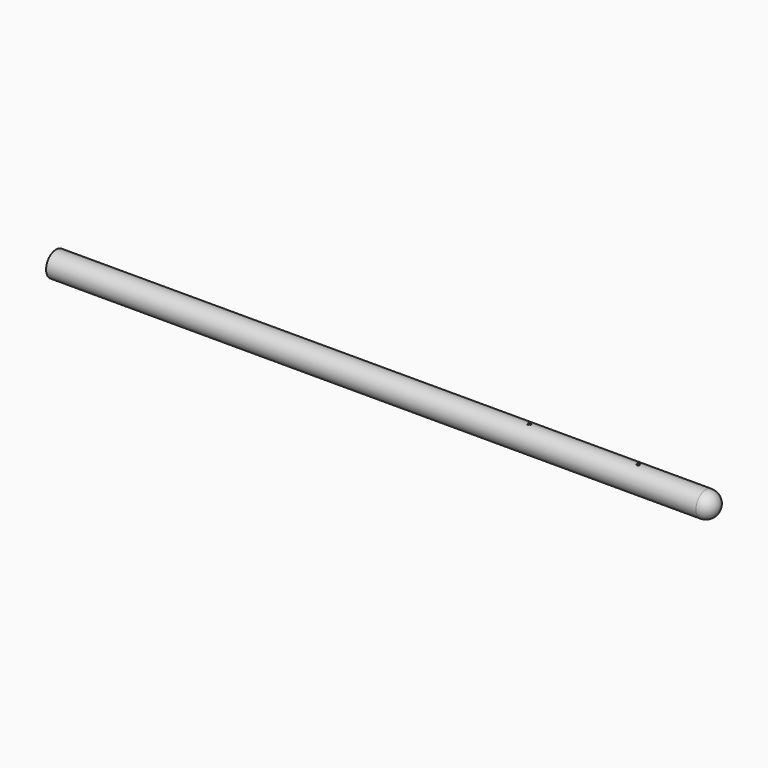
from build123d import *

# Parameters (mm, degrees)
F2_T      = -12.7
F3_R      = 50.8
F4_DEPTH  = 254
F5_DEPTH  = 25.4
F6_R      = 12.7
F7_DEPTH  = 304.8
F9_R      = 15.0991229188
F9_R_2    = 6.35
F9_R_3    = 14.3550520621
F10_DEPTH = 12.7
F11_R     = 5.08
F12_SIZE  = 1.27
F13_R     = 5.08


with BuildPart() as f1:
    # F0 (on Front) → F1 (revolve)
    with BuildSketch(Plane.XZ):
        with BuildLine():
            Line((0, 152.4), (0, 0))
            Line((0, 0), (7924.8, 0))
            Line((7924.8, 0), (8077.2, 0))
            ThreePointArc((8077.2, 0), (8032.5630734528, 107.7630734528), (7924.8, 152.4))
            Line((7924.8, 152.4), (0, 152.4))
        make_face()
    revolve(axis=Axis((4038.6, 0, 0), (1, 0, 0)))

    # F2
    f2_openings = [f1.faces().sort_by_distance(p)[0] for p in [
        (0, 0, 0),
    ]]
    offset(amount=F2_T, openings=f2_openings)

    # F3 (on Top) → F4 (cut)
    with BuildSketch(Plane.XY):
        with Locations((7620, 0)):
            Circle(F3_R)
        with Locations((6096, 0)):
            Circle(F3_R)
        with Locations((4572, 0)):
            Circle(F3_R)
        with Locations((3048, 0)):
            Circle(F3_R)
        with Locations((1524, 0)):
            Circle(F3_R)
    extrude(amount=-F4_DEPTH, mode=Mode.SUBTRACT)

    # F6 (on Top) → F7 (cut)
    with BuildSketch(Plane.XY):
        with Locations((7100.4438400269, 0)):
            Circle(F6_R)
        with Locations((5773.1170654297, 0)):
            Circle(F6_R)
    extrude(amount=F7_DEPTH, mode=Mode.SUBTRACT)

    # F9 (on offset) → F10 (join, symmetric)
    with BuildSketch(Plane.XY.offset(152.4)):
        with Locations((5772.6697921753, 0)):
            Circle(F9_R)
        with Locations((5772.6697921753, 0)):
            Circle(F9_R_2, mode=Mode.SUBTRACT)
        with Locations((7100.5816459656, 0)):
            Circle(F9_R_3)
        with Locations((7100.5816459656, 0)):
            Circle(F9_R_2, mode=Mode.SUBTRACT)
    extrude(amount=F10_DEPTH, both=True)

    # F11
    f11_edges = [f1.edges().sort_by_distance(p)[0] for p in [
        (7100.581646, -14.355052, 151.722419),
        (7100.581646, 14.355052, 151.722419),
    ]]
    fillet(f11_edges, radius=F11_R)

    # F12
    f12_edges = [f1.edges().sort_by_distance(p)[0] for p in [
        (7086.226594, 0, 165.1),
        (5757.570669, 0, 165.1),
    ]]
    chamfer(f12_edges, length=F12_SIZE)

    # F13
    f13_edges = [f1.edges().sort_by_distance(p)[0] for p in [
        (5772.669792, -15.099123, 151.650178),
        (5772.669792, 15.099123, 151.650178),
    ]]
    fillet(f13_edges, radius=F13_R)


with BuildPart() as f5:
    # F3 (on Top) → F5 (new body)
    with BuildSketch(Plane.XY):
        with Locations((7620, 0)):
            Circle(F3_R)
    extrude(amount=F5_DEPTH)


with BuildPart() as f5b:
    # F3 (on Top) → F5, piece 2 (new body)
    with BuildSketch(Plane.XY):
        with Locations((6096, 0)):
            Circle(F3_R)
    extrude(amount=F5_DEPTH)


with BuildPart() as f5c:
    # F3 (on Top) → F5, piece 3 (new body)
    with BuildSketch(Plane.XY):
        with Locations((4572, 0)):
            Circle(F3_R)
    extrude(amount=F5_DEPTH)


with BuildPart() as f5d:
    # F3 (on Top) → F5, piece 4 (new body)
    with BuildSketch(Plane.XY):
        with Locations((3048, 0)):
            Circle(F3_R)
    extrude(amount=F5_DEPTH)


with BuildPart() as f5e:
    # F3 (on Top) → F5, piece 5 (new body)
    with BuildSketch(Plane.XY):
        with Locations((1524, 0)):
            Circle(F3_R)
    extrude(amount=F5_DEPTH)


solid = Compound([f1.part, f5.part, f5b.part, f5c.part, f5d.part, f5e.part])
